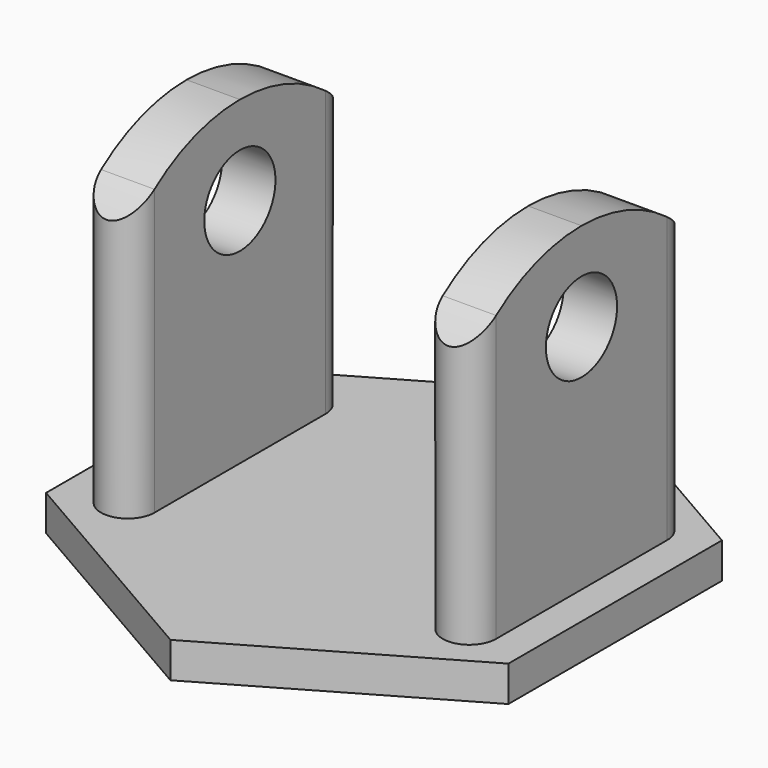
from build123d import *

# Parameters (mm, degrees)
F1_DEPTH = 10
F3_DEPTH = 90
F4_R     = 12.5
F5_DEPTH = 120.4529052838


# Not quite as in the source:
# - a pattern or mirror of a feature is missing from the dataset's text; its kind, count and spacing are read off the source's solid


with BuildPart() as f1:
    # F0 (on Top) → F1 (new body)
    with BuildSketch(Plane.XY):
        Polygon((-64.9519052838, -37.5), (0, -75), (64.9519052838, -37.5), (64.9519052838, 37.5), (0, 75), (-64.9519052838, 37.5), align=None)
    extrude(amount=F1_DEPTH)

    # F2 (on face) → F3 (join)
    with BuildSketch(Plane.XY.offset(10)):
        with BuildLine():
            Line((-40.5, -30), (-40.5, 0))
            ThreePointArc((-40.5, 0), (-48, -7.5), (-55.5, 0))
            Line((-55.5, 0), (-55.5, -30))
            ThreePointArc((-55.5, -30), (-48, -37.5), (-40.5, -30))
        make_face()
        with BuildLine():
            ThreePointArc((-55.5, 0), (-48, -7.5), (-40.5, 0))
            ThreePointArc((-40.5, 0), (-48, 7.5), (-55.5, 0))
        make_face()
        with BuildLine():
            ThreePointArc((-55.5, 0), (-48, 7.5), (-40.5, 0))
            Line((-40.5, 0), (-40.5, 30))
            ThreePointArc((-40.5, 30), (-48, 37.5), (-55.5, 30))
            Line((-55.5, 30), (-55.5, 0))
        make_face()
    f3 = extrude(amount=F3_DEPTH)

    # F3_copies: F3 across plane
    add(f3.mirror(Plane(origin=(0, 0, 0), x_dir=(0, 0, 1), z_dir=(1, 0, 0))))

    # F4 (on face) → F5 (cut, through all)
    with BuildSketch(Plane(origin=(-55.5, 0, 0), x_dir=(0, -1, 0), z_dir=(-1, 0, 0))):
        with BuildLine():
            ThreePointArc((-38, 82.4961536185), (-34.2063872344, 86.4681103482), (-30, 90))
            Line((-30, 90), (-30, 100))
            Line((-30, 100), (-38, 100))
            Line((-38, 100), (-38, 82.4961536185))
        make_face()
        with BuildLine():
            ThreePointArc((-30, 90), (-15.8113883008, 97.4341649025), (0, 100))
            Line((0, 100), (-30, 100))
            Line((-30, 100), (-30, 90))
        make_face()
        with BuildLine():
            ThreePointArc((0, 100), (15.8113883008, 97.4341649025), (30, 90))
            Line((30, 90), (30, 100))
            Line((30, 100), (0, 100))
        make_face()
        with BuildLine():
            ThreePointArc((30, 90), (34.2063872344, 86.4681103482), (38, 82.4961536185))
            Line((38, 82.4961536185), (38, 100))
            Line((38, 100), (30, 100))
            Line((30, 100), (30, 90))
        make_face()
        with Locations((0, 75)):
            Circle(F4_R)
    extrude(amount=-F5_DEPTH, mode=Mode.SUBTRACT)


solid = f1.part
